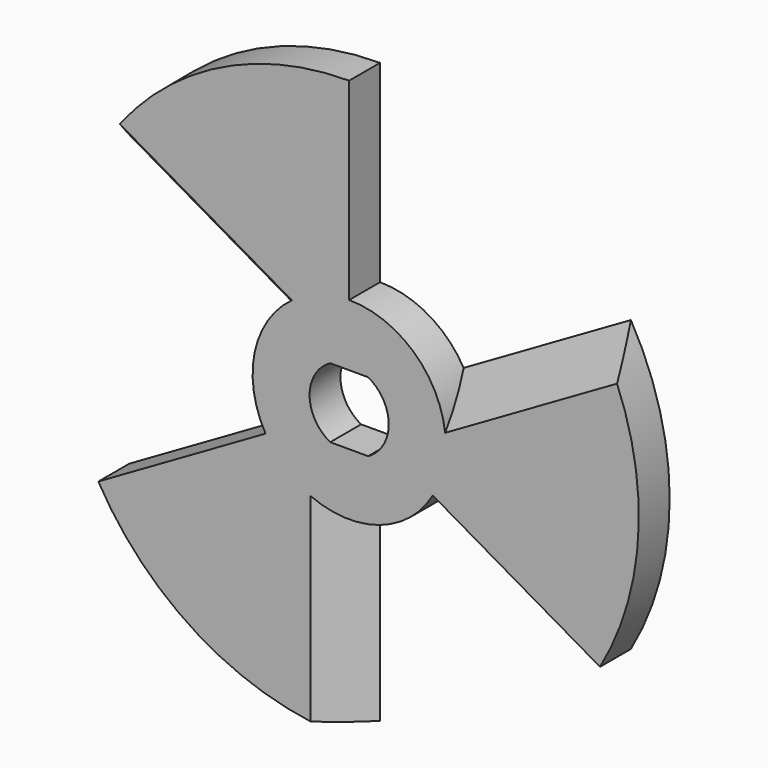
from build123d import *

# Parameters (mm, degrees)
F1_DEPTH = 20
F2_SIZE  = 19.99999


# Not quite as in the source:
# - a fillet or chamfer is up to 0.001 mm smaller than in the source, because OpenCascade refuses the exact size


with BuildPart() as f1:
    # F0 (on Front) → F1 (new body)
    with BuildSketch(Plane.XZ):
        with BuildLine():
            Line((-129.9038105677, 75), (-43.3012701892, 25))
            ThreePointArc((-43.3012701892, 25), (-50, 0), (-43.3012701892, -25))
            Line((-43.3012701892, -25), (-129.9038105677, -75))
            ThreePointArc((-129.9038105677, -75), (-75, -129.9038105677), (0, -150))
            Line((0, -150), (0, -50))
            ThreePointArc((0, -50), (25, -43.3012701892), (43.3012701892, -25))
            Line((43.3012701892, -25), (129.9038105677, -75))
            ThreePointArc((129.9038105677, -75), (150, 0), (129.9038105677, 75))
            Line((129.9038105677, 75), (43.3012701892, 25))
            ThreePointArc((43.3012701892, 25), (25, 43.3012701892), (0, 50))
            Line((0, 50), (0, 150))
            ThreePointArc((0, 150), (-75, 129.9038105677), (-129.9038105677, 75))
        make_face()
        with BuildLine():
            ThreePointArc((-9.8107084352, -18), (-20.5, 0), (-9.8107084352, 18))
            Line((-9.8107084352, 18), (9.8107084352, 18))
            ThreePointArc((9.8107084352, 18), (20.5, 0), (9.8107084352, -18))
            Line((9.8107084352, -18), (-9.8107084352, -18))
        make_face(mode=Mode.SUBTRACT)
    extrude(amount=F1_DEPTH)

    # F2 (size 20 in the source; OpenCascade refuses exactly that, so slightly less here)
    f2_edges = [f1.edges().sort_by_distance(p)[0] for p in [
        (-86.60254, -20, 50),
        (0, -20, -100),
        (86.60254, -20, 50),
    ]]
    chamfer(f2_edges, length=F2_SIZE)


solid = f1.part
